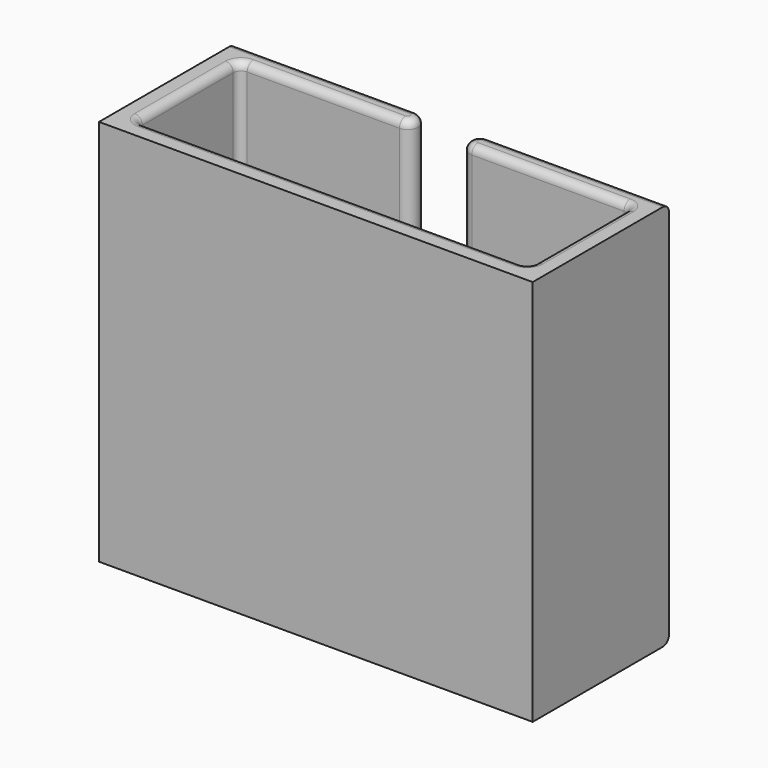
from build123d import *

# Parameters (mm, degrees)
F1_DEPTH = 75
F2_F1_R  = 1.5
F2_F2_R  = 1.5
F4_W     = 18
F4_H     = 55
F5_DEPTH = 0.5


# Not quite as in the source:
# - a feature names something its author has since deleted; it is built from what else it names


with BuildPart() as f1:
    # F0 (on Top) → F1 (new body)
    with BuildSketch(Plane.XY):
        with BuildLine():
            Line((38, 12.5), (38, -12.5))
            Line((38, -12.5), (-38, -12.5))
            Line((-38, -12.5), (-38, 12.5))
            Line((-38, 12.5), (-7, 12.5))
            ThreePointArc((-7, 12.5), (-5, 14.5), (-7, 16.5))
            Line((-7, 16.5), (-42, 16.5))
            Line((-42, 16.5), (-42, -16.5))
            Line((-42, -16.5), (42, -16.5))
            Line((42, -16.5), (42, 16.5))
            Line((42, 16.5), (7, 16.5))
            ThreePointArc((7, 16.5), (5, 14.5), (7, 12.5))
            Line((7, 12.5), (38, 12.5))
        make_face()
    extrude(amount=F1_DEPTH)

    # F2: fillet of radius 1.5 on 12 edges, made by hand

    # F2_f1
    f2_f1_edges = [f1.edges().sort_by_distance(p)[0] for p in [
        (38, -12.5, 37.5),
        (-38, -12.5, 37.5),
        (-38, 12.5, 37.5),
        (38, 12.5, 37.5),
    ]]
    fillet(f2_f1_edges, radius=F2_F1_R)

    # F2_f2
    f2_f2_edges = [f1.edges().sort_by_distance(p)[0] for p in [
        (0, -12.5, 0),
        (0, -12.5, 75),
        (21.75, 12.5, 0),
        (21.75, 12.5, 75),
        (5, 14.5, 75),
        (24.5, 16.5, 75),
        (5, 14.5, 0),
        (24.5, 16.5, 0),
        (37.5606601718, 12.0606601718, 75),
        (37.5606601718, 12.0606601718, 0),
        (37.5606601718, -12.0606601718, 75),
        (-37.5606601718, -12.0606601718, 75),
        (37.5606601718, -12.0606601718, 0),
        (-37.5606601718, -12.0606601718, 0),
    ]]
    fillet(f2_f2_edges, radius=F2_F2_R)

    # F4 (on offset) → F5 (cut)
    with BuildSketch(Plane(origin=(0, 16.5, 0), x_dir=(-1, 0, 0), z_dir=(0, 1, 0))):
        with Locations((-24.5, 47.5)):
            Rectangle(F4_W, F4_H)
        with Locations((24.5, 47.5)):
            Rectangle(F4_W, F4_H)
    extrude(amount=-F5_DEPTH, mode=Mode.SUBTRACT)


solid = f1.part
